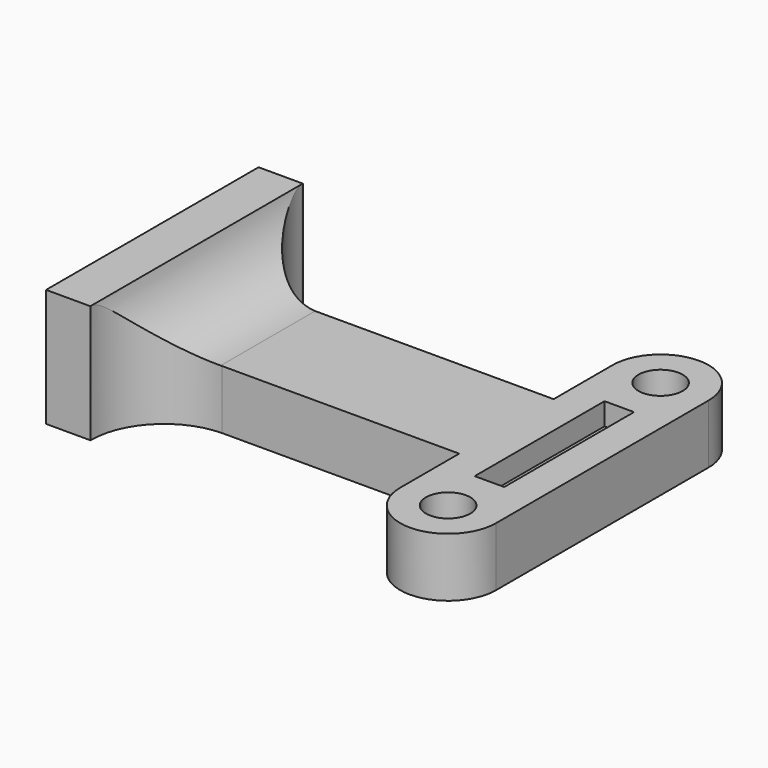
from build123d import *

# Parameters (mm, degrees)
F0_R         = 1.5
F0_W         = 21
F0_H         = 8
F0_W_2       = 3
F0_H_2       = 5
F1_DEPTH     = 4
F2_W         = 2
F2_H         = 11
F3_DEPTH     = 1.5
F4_DEPTH     = 8
F5_T1_DEPTH  = 4
F5_T3_DEPTH  = 8
F5_T9_DEPTH  = 20.2494197933
F5_T14_DEPTH = 16.5024140205
F5_T22_DEPTH = 20.2494197933
F5_T27_DEPTH = 16.5024140205


# Not quite as in the source:
# - a fillet or chamfer that OpenCascade refuses, or shapes differently, is made with other operations: its cross-section is extruded or revolved along the edge and cut away or added


with BuildPart() as f1:
    # F0 (on Top) → F1 (new body)
    with BuildSketch(Plane.XY):
        with BuildLine():
            ThreePointArc((-3.25, 9), (0, 5.75), (3.25, 9))
            ThreePointArc((3.25, 9), (0, 12.25), (-3.25, 9))
        make_face()
        with Locations((0, 9)):
            Circle(F0_R, mode=Mode.SUBTRACT)
        with BuildLine():
            Line((3.25, -9), (3.25, 9))
            ThreePointArc((3.25, 9), (0, 5.75), (-3.25, 9))
            Line((-3.25, 9), (-3.25, 4))
            Line((-3.25, 4), (-3.25, -4))
            Line((-3.25, -4), (-3.25, -9))
            ThreePointArc((-3.25, -9), (0, -5.75), (3.25, -9))
        make_face()
        with BuildLine():
            ThreePointArc((-3.25, -9), (0, -12.25), (3.25, -9))
            ThreePointArc((3.25, -9), (0, -5.75), (-3.25, -9))
        make_face()
        with Locations((0, -9)):
            Circle(F0_R, mode=Mode.SUBTRACT)
        with Locations((-13.75, 0)):
            Rectangle(F0_W, F0_H)
        with Locations((-25.75, 0)):
            Rectangle(F0_W_2, F0_H)
        with Locations((-25.75, 6.5)):
            Rectangle(F0_W_2, F0_H_2)
        with Locations((-25.75, -6.5)):
            Rectangle(F0_W_2, F0_H_2)
    extrude(amount=F1_DEPTH)

    # F2 (on face) → F3 (cut)
    with BuildSketch(Plane.XY.offset(4)):
        Rectangle(F2_W, F2_H)
    extrude(amount=-F3_DEPTH, mode=Mode.SUBTRACT)

    # F0 (on Top) → F4 (join)
    with BuildSketch(Plane.XY):
        with Locations((-25.75, 6.5)):
            Rectangle(F0_W_2, F0_H_2)
        with Locations((-25.75, 0)):
            Rectangle(F0_W_2, F0_H)
        with Locations((-25.75, -6.5)):
            Rectangle(F0_W_2, F0_H_2)
    extrude(amount=F4_DEPTH)

    # F5: fillet of radius 5 on 3 edges, made by hand

    # F5_s2 → F5_t1 (join)
    with BuildSketch(Plane.XY):
        with BuildLine():
            ThreePointArc((-19.2490344078, 3.9996), (-22.785192534, 5.4641246619), (-24.2504, 8.9999999228))
            Line((-24.2504, 8.9999999228), (-24.7505365592, 8.9999033465))
            ThreePointArc((-24.7505365592, 8.9999033465), (-24.7501365685, 6.4999999614), (-24.7501365685, 4))
            Line((-24.7501365685, 4), (-24.25, 3.4998634315))
            ThreePointArc((-24.25, 3.4998634315), (-21.7495172039, 3.4998634315), (-19.2490344078, 3.4994634315))
            Line((-19.2490344078, 3.4994634315), (-19.2490344078, 3.9996))
        make_face()
        with BuildLine():
            ThreePointArc((-24.2504, -8.9999999228), (-22.785192534, -5.4641246619), (-19.2490344078, -3.9996))
            Line((-19.2490344078, -3.9996), (-19.2490344078, -3.4994634315))
            ThreePointArc((-19.2490344078, -3.4994634315), (-21.7495172039, -3.4998634315), (-24.25, -3.4998634315))
            Line((-24.25, -3.4998634315), (-24.7501365685, -4))
            ThreePointArc((-24.7501365685, -4), (-24.7501365685, -6.4999999614), (-24.7505365592, -8.9999033465))
            Line((-24.7505365592, -8.9999033465), (-24.2504, -8.9999999228))
        make_face()
    extrude(amount=F5_T1_DEPTH)

    # F5_s4 → F5_t3 (join)
    with BuildSketch(Plane.XZ.offset(-4)):
        with BuildLine():
            ThreePointArc((-19.350232099, 3.9996), (-22.5130680788, 5.126675133), (-24.2503919057, 7.9999199382))
            Line((-24.2503919057, 7.9999199382), (-24.7404078864, 7.8998153635))
            ThreePointArc((-24.7404078864, 7.8998153635), (-24.7501365685, 5.9999599691), (-24.7501365685, 4))
            Line((-24.7501365685, 4), (-24.25, 3.4998634315))
            ThreePointArc((-24.25, 3.4998634315), (-21.8001160495, 3.4998634315), (-19.350232099, 3.4994634315))
            Line((-19.350232099, 3.4994634315), (-19.350232099, 3.9996))
        make_face()
    extrude(amount=F5_T3_DEPTH)


with BuildPart() as f5_tool7:
    # F5_s8 → F5_t9 (new body)
    with BuildSketch(Plane.XZ.offset(-16.2494197933)):
        with BuildLine():
            ThreePointArc((-19.350232099, 3.9996), (-22.5130680788, 5.126675133), (-24.2503919057, 7.9999199382))
            Line((-24.2503919057, 7.9999199382), (-24.7404078864, 7.8998153635))
            ThreePointArc((-24.7404078864, 7.8998153635), (-24.7501365685, 5.9999599691), (-24.7501365685, 4))
            Line((-24.7501365685, 4), (-24.25, 3.4998634315))
            ThreePointArc((-24.25, 3.4998634315), (-21.8001160495, 3.4998634315), (-19.350232099, 3.4994634315))
            Line((-19.350232099, 3.4994634315), (-19.350232099, 3.9996))
        make_face()
    extrude(amount=F5_T9_DEPTH)

    split(bisect_by=Plane.XZ.offset(-4), keep=Keep.BOTTOM)

    split(bisect_by=Plane.XZ.offset(-9), keep=Keep.TOP)


with BuildPart() as f5_tool12:
    # F5_s13 → F5_t14 (new body)
    with BuildSketch(Plane.XY):
        with BuildLine():
            ThreePointArc((-19.2490344078, 3.9996), (-22.785192534, 5.4641246619), (-24.2504, 8.9999999228))
            Line((-24.2504, 8.9999999228), (-24.7505365592, 8.9999033465))
            ThreePointArc((-24.7505365592, 8.9999033465), (-24.7501365685, 6.4999999614), (-24.7501365685, 4))
            Line((-24.7501365685, 4), (-24.25, 3.4998634315))
            ThreePointArc((-24.25, 3.4998634315), (-21.7495172039, 3.4998634315), (-19.2490344078, 3.4994634315))
            Line((-19.2490344078, 3.4994634315), (-19.2490344078, 3.9996))
        make_face()
    extrude(amount=F5_T14_DEPTH)

    split(bisect_by=Plane.XY.offset(4), keep=Keep.TOP)

    split(bisect_by=Plane.XY.offset(8), keep=Keep.BOTTOM)


with BuildPart() as f5_tool7_1:
    add(f5_tool7.part)

    # F5_t17: intersect F5_tool12
    add(f5_tool12.part, mode=Mode.INTERSECT)


with BuildPart() as f1_1:
    add(f1.part)

    # F5_t5: union F5_tool7
    add(f5_tool7_1.part)


with BuildPart() as f5_tool20:
    # F5_s21 → F5_t22 (new body)
    with BuildSketch(Plane.XZ.offset(-4)):
        with BuildLine():
            ThreePointArc((-19.350232099, 3.9996), (-22.5130680788, 5.126675133), (-24.2503919057, 7.9999199382))
            Line((-24.2503919057, 7.9999199382), (-24.7404078864, 7.8998153635))
            ThreePointArc((-24.7404078864, 7.8998153635), (-24.7501365685, 5.9999599691), (-24.7501365685, 4))
            Line((-24.7501365685, 4), (-24.25, 3.4998634315))
            ThreePointArc((-24.25, 3.4998634315), (-21.8001160495, 3.4998634315), (-19.350232099, 3.4994634315))
            Line((-19.350232099, 3.4994634315), (-19.350232099, 3.9996))
        make_face()
    extrude(amount=F5_T22_DEPTH)

    split(bisect_by=Plane.XZ.offset(9), keep=Keep.BOTTOM)

    split(bisect_by=Plane.XZ.offset(4), keep=Keep.TOP)


with BuildPart() as f5_tool25:
    # F5_s26 → F5_t27 (new body)
    with BuildSketch(Plane.XY):
        with BuildLine():
            ThreePointArc((-24.2504, -8.9999999228), (-22.785192534, -5.4641246619), (-19.2490344078, -3.9996))
            Line((-19.2490344078, -3.9996), (-19.2490344078, -3.4994634315))
            ThreePointArc((-19.2490344078, -3.4994634315), (-21.7495172039, -3.4998634315), (-24.25, -3.4998634315))
            Line((-24.25, -3.4998634315), (-24.7501365685, -4))
            ThreePointArc((-24.7501365685, -4), (-24.7501365685, -6.4999999614), (-24.7505365592, -8.9999033465))
            Line((-24.7505365592, -8.9999033465), (-24.2504, -8.9999999228))
        make_face()
    extrude(amount=F5_T27_DEPTH)

    split(bisect_by=Plane.XY.offset(4), keep=Keep.TOP)

    split(bisect_by=Plane.XY.offset(8), keep=Keep.BOTTOM)


with BuildPart() as f5_tool20_1:
    add(f5_tool20.part)

    # F5_t30: intersect F5_tool25
    add(f5_tool25.part, mode=Mode.INTERSECT)


with BuildPart() as f1_2:
    add(f1_1.part)

    # F5_t18: union F5_tool20
    add(f5_tool20_1.part)


solid = f1_2.part
